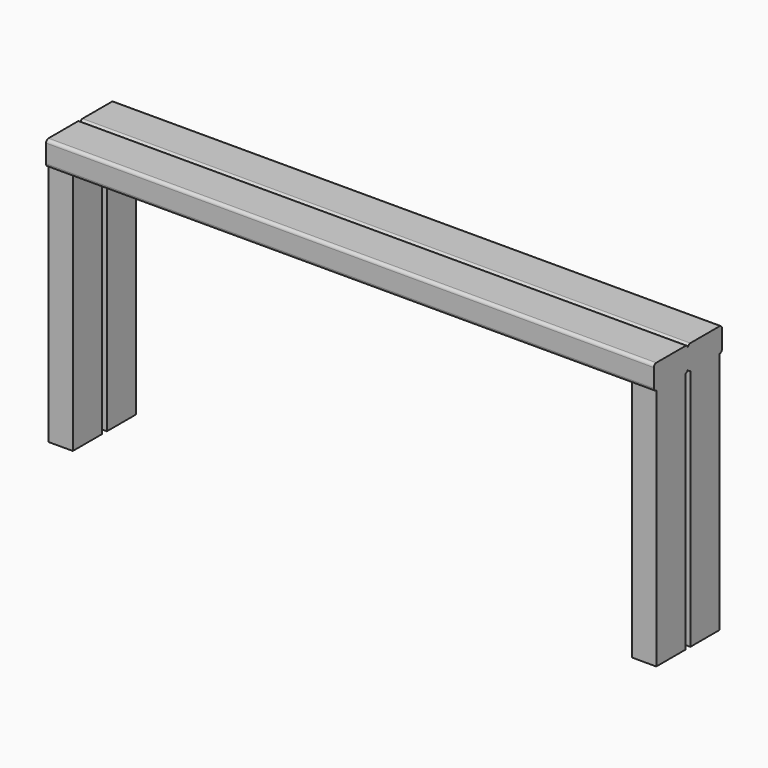
from build123d import *

# Parameters (mm, degrees)
F1_DEPTH = 500
F2_W     = 40
F2_H     = 60
F3_DEPTH = 400


# Not quite as in the source:
# - a pattern or mirror of a feature is missing from the dataset's text; its kind, count and spacing are read off the source's solid


with BuildPart() as f1:
    # F0 (on Right) → F1 (new body, symmetric)
    with BuildSketch(Plane.YZ):
        with BuildLine():
            Line((-65, 0), (-5, 0))
            ThreePointArc((-5, 0), (-1.4644660941, 1.4644660941), (0, 5))
            Line((0, 5), (0, 35))
            ThreePointArc((0, 35), (-1.4644660941, 38.5355339059), (-5, 40))
            Line((-5, 40), (-65, 40))
            ThreePointArc((-65, 40), (-68.5355339059, 38.5355339059), (-70, 35))
            Line((-70, 35), (-70, 5))
            ThreePointArc((-70, 5), (-68.5355339059, 1.4644660941), (-65, 0))
        make_face()
    extrude(amount=F1_DEPTH, both=True)

    # F2 (on face) → F3 (join)
    with BuildSketch(Plane(origin=(0, 0, 0), x_dir=(1, 0, 0), z_dir=(0, 0, -1))):
        with Locations((480, 35)):
            Rectangle(F2_W, F2_H)
    f3 = extrude(amount=F3_DEPTH)

    # F3_copies: F3 across plane
    add(f3.mirror(Plane(origin=(0, 0, 0), x_dir=(0, 0, -1), z_dir=(-1, 0, 0))))

    # F4: F1 across plane


with BuildPart() as f1_1:
    add(f1.part)
    add(f1.part.mirror(Plane.XZ))


solid = f1_1.part
